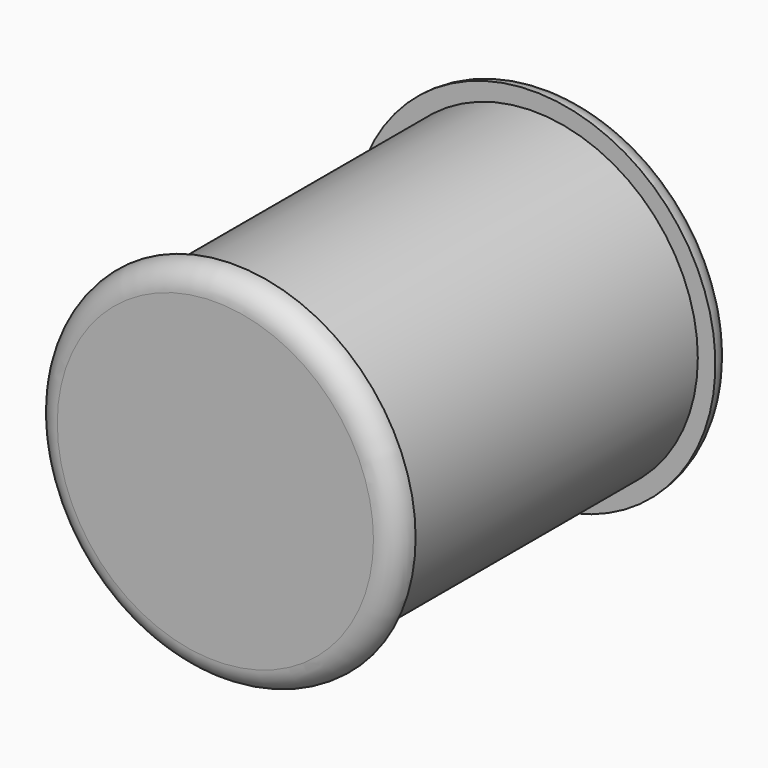
from build123d import *

# Parameters (mm, degrees)
F0_R     = 7
F1_DEPTH = 8
F2_R     = 7.75
F2_R_2   = 7
F3_DEPTH = 1
F4_R     = 7.75
F4_R_2   = 7
F5_DEPTH = 1
F6_R     = 0.99999


# Not quite as in the source:
# - a fillet or chamfer is up to 0.001 mm smaller than in the source, because OpenCascade refuses the exact size


with BuildPart() as f1:
    # F0 (on Front) → F1 (new body, symmetric)
    with BuildSketch(Plane.XZ):
        Circle(F0_R)
    extrude(amount=F1_DEPTH, both=True)

    # F2 (on face) → F3 (join)
    with BuildSketch(Plane.XZ.offset(8)):
        Circle(F2_R)
        Circle(F2_R_2, mode=Mode.SUBTRACT)
        Circle(F2_R_2)
    extrude(amount=F3_DEPTH)

    # F4 (on face) → F5 (join)
    with BuildSketch(Plane(origin=(0, 8, 0), x_dir=(-1, 0, 0), z_dir=(0, 1, 0))):
        Circle(F4_R)
        Circle(F4_R_2, mode=Mode.SUBTRACT)
        Circle(F4_R_2)
    extrude(amount=F5_DEPTH)

    # F6 (radius 1 in the source; OpenCascade refuses exactly that, so slightly less here)
    f6_edges = [f1.edges().sort_by_distance(p)[0] for p in [
        (-7.75, -9, 0),
        (7.75, 9, 0),
    ]]
    fillet(f6_edges, radius=F6_R)


solid = f1.part
